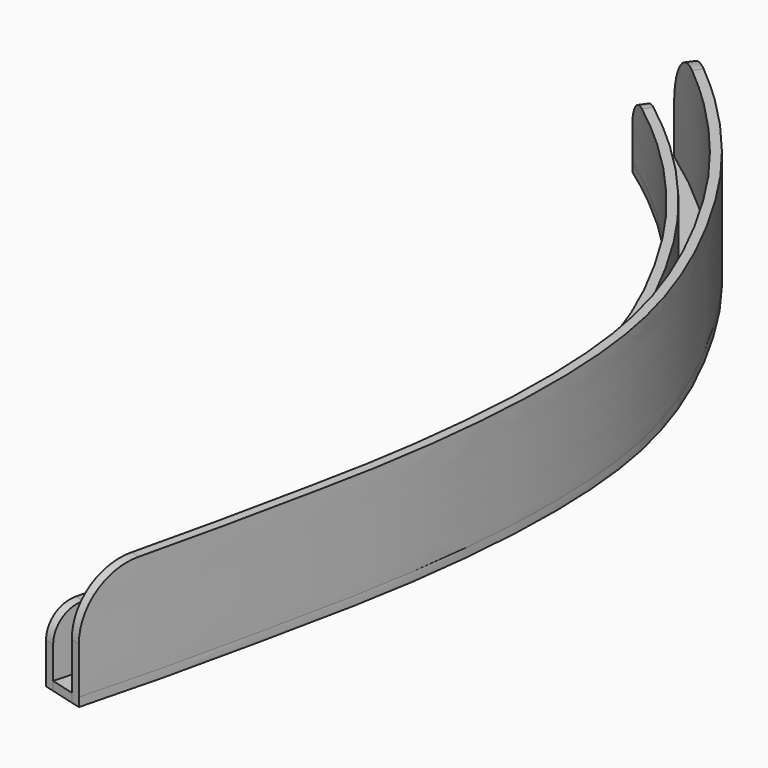
from build123d import *

# Parameters (mm, degrees)
F1_DEPTH = 1.5
F2_DEPTH = 12
F3_DEPTH = 19.5
F4_R     = 5
F5_R     = 10


# Not quite as in the source:
# - the dataset's text gives a spline's control points without its knots; the knots are read off the source's solid


with BuildPart() as f1:
    # F0 (on Top) → F1 (new body)
    with BuildSketch(Plane.XY):
        with BuildLine():
            Line((-5.5994206801, 1.5121137679), (-4.0547529063, 1.0949789353))
            add(Edge.make_bspline(
                [(-4.0547529063, 1.0949789353), (-2.7584482404, 5.8952494629), (-0.507776567, 14.8690865032), (1.6924327705, 24.7406730259), (3.2274659258, 31.9644086425), (4.3072829593, 37.0843203018), (5.3299777431, 41.9138704286), (6.2857824418, 46.6537900391), (7.0272963269, 50.6976340906), (7.5873908522, 54.0943139859), (7.9908458474, 56.7487025574), (8.3776794398, 59.5373035181), (8.7470381673, 62.4820190039), (9.0884901288, 65.5597847369), (9.4935897179, 69.8161894419), (9.8812175689, 75.3734994318), (10.0786737767, 82.263177237), (9.9568653112, 88.0547624157), (9.6514350357, 92.6366085021), (9.3098136977, 96.0260880656), (8.8477649235, 99.3496211049), (8.2569195036, 102.5793684142), (7.5320301271, 105.7399534193), (6.4089069299, 109.8549418842), (4.7452423063, 114.7999787819), (2.4491955615, 120.3732711408), (0.3841711701, 124.6808678941), (-1.2995078927, 127.9041144647), (-2.5628466606, 130.2043090367), (-3.8134120185, 132.3855904729), (-5.0303692601, 134.4303909952), (-6.225751369, 136.3562424102), (-7.8102832693, 138.7970536423), (-9.4097420041, 141.0929548178), (-11.0855205079, 143.3377393291), (-12.3960339805, 145.0187641433), (-13.7763443543, 146.7201318409), (-15.72650292, 149.0430807319), (-18.3677148559, 152.0208171993), (-21.9677844701, 155.7272991211), (-27.4687288943, 160.8505391151), (-32.5300323602, 164.9012591785), (-36.4483448757, 167.6911563366)],
                knots=[0, 0, 0, 0, 0.0625, 0.125, 0.15625, 0.1875, 0.21875, 0.25, 0.28125, 0.296875, 0.3125, 0.328125, 0.34375, 0.359375, 0.375, 0.40625, 0.4375, 0.46875, 0.484375, 0.5, 0.515625, 0.53125, 0.546875, 0.5625, 0.59375, 0.625, 0.65625, 0.671875, 0.6875, 0.703125, 0.71875, 0.734375, 0.75, 0.78125, 0.796875, 0.8125, 0.828125, 0.84375, 0.875, 0.90625, 0.9375, 1, 1, 1, 1], degree=3))
            Line((-36.4483448757, 167.6911563366), (-37.3763651787, 166.3877844337))
            add(Edge.make_bspline(
                [(-5.5994206801, 1.5121137679), (-4.3077783691, 6.2951193997), (-2.6258306552, 13.0012722172), (-0.7487467422, 21.1428564548), (0.5120539371, 26.8835227425), (1.6618421424, 32.2942963304), (2.7421119556, 37.4163284129), (3.763711516, 42.2407810647), (4.7148473297, 46.957842903), (5.4512317261, 50.973867239), (6.0070554882, 54.3446698739), (6.4074062474, 56.9786211877), (6.7913909073, 59.7466701592), (7.1580594369, 62.6699482968), (7.4968679186, 65.7239423227), (7.8986708212, 69.9457663896), (8.2827863792, 75.4536557983), (8.4780584917, 82.2716892525), (8.3575613015, 87.9906565389), (8.0566182326, 92.5041987263), (7.7206413282, 95.8370668347), (7.2673362217, 99.0969692413), (6.6893645236, 102.2561266917), (5.9799138442, 105.3495938294), (4.8790699069, 109.3831785269), (3.2460371404, 114.2377292155), (0.9873722214, 119.7207845936), (-1.0479591133, 123.9666951238), (-2.7098338186, 127.1482330689), (-3.9579699642, 129.4207865652), (-5.1952414945, 131.578886851), (-6.3982341438, 133.6001882211), (-7.5769680108, 135.4991721914), (-9.137149923, 137.90242787), (-10.7091151944, 140.1588272478), (-12.3574452199, 142.3668701842), (-13.6477758322, 144.0220399555), (-15.010114653, 145.7012846996), (-16.4552376121, 147.422652176), (-17.9785130359, 149.1706475813), (-20.1319914125, 151.5406139455), (-23.0870853339, 154.5830386116), (-28.5072460687, 159.6311117942), (-33.5019044586, 163.6291104104), (-37.3763651787, 166.3877844337)],
                knots=[0, 0, 0, 0, 0.0625, 0.09375, 0.125, 0.15625, 0.1875, 0.21875, 0.25, 0.28125, 0.296875, 0.3125, 0.328125, 0.34375, 0.359375, 0.375, 0.40625, 0.4375, 0.46875, 0.484375, 0.5, 0.515625, 0.53125, 0.546875, 0.5625, 0.59375, 0.625, 0.65625, 0.671875, 0.6875, 0.703125, 0.71875, 0.734375, 0.75, 0.78125, 0.796875, 0.8125, 0.828125, 0.84375, 0.859375, 0.875, 0.90625, 0.9375, 1, 1, 1, 1], degree=3))
        make_face()
        with BuildLine():
            Line((-4.0547529063, 1.0949789353), (0, 0))
            add(Edge.make_bspline(
                [(0, 0), (3.7575578317, 13.9143941924), (8.0227826013, 34.5697242327), (13.2830483989, 58.810255219), (16.3286613818, 102.3745951935), (0.7414565413, 134.1840402305), (-10.850321997, 150.6677651162), (-23.166189723, 163.3899207212), (-34.0122915804, 171.1125075817)],
                knots=[0, 0, 0, 0, 0.179472721, 0.3278596656, 0.5244539041, 0.7009046035, 0.8319408255, 1, 1, 1, 1], degree=3))
            Line((-34.0122915804, 171.1125075817), (-36.4483448757, 167.6911563366))
            add(Edge.make_bspline(
                [(-4.0547529063, 1.0949789353), (-2.7584482404, 5.8952494629), (-0.507776567, 14.8690865032), (1.6924327705, 24.7406730259), (3.2274659258, 31.9644086425), (4.3072829593, 37.0843203018), (5.3299777431, 41.9138704286), (6.2857824418, 46.6537900391), (7.0272963269, 50.6976340906), (7.5873908522, 54.0943139859), (7.9908458474, 56.7487025574), (8.3776794398, 59.5373035181), (8.7470381673, 62.4820190039), (9.0884901288, 65.5597847369), (9.4935897179, 69.8161894419), (9.8812175689, 75.3734994318), (10.0786737767, 82.263177237), (9.9568653112, 88.0547624157), (9.6514350357, 92.6366085021), (9.3098136977, 96.0260880656), (8.8477649235, 99.3496211049), (8.2569195036, 102.5793684142), (7.5320301271, 105.7399534193), (6.4089069299, 109.8549418842), (4.7452423063, 114.7999787819), (2.4491955615, 120.3732711408), (0.3841711701, 124.6808678941), (-1.2995078927, 127.9041144647), (-2.5628466606, 130.2043090367), (-3.8134120185, 132.3855904729), (-5.0303692601, 134.4303909952), (-6.225751369, 136.3562424102), (-7.8102832693, 138.7970536423), (-9.4097420041, 141.0929548178), (-11.0855205079, 143.3377393291), (-12.3960339805, 145.0187641433), (-13.7763443543, 146.7201318409), (-15.72650292, 149.0430807319), (-18.3677148559, 152.0208171993), (-21.9677844701, 155.7272991211), (-27.4687288943, 160.8505391151), (-32.5300323602, 164.9012591785), (-36.4483448757, 167.6911563366)],
                knots=[0, 0, 0, 0, 0.0625, 0.125, 0.15625, 0.1875, 0.21875, 0.25, 0.28125, 0.296875, 0.3125, 0.328125, 0.34375, 0.359375, 0.375, 0.40625, 0.4375, 0.46875, 0.484375, 0.5, 0.515625, 0.53125, 0.546875, 0.5625, 0.59375, 0.625, 0.65625, 0.671875, 0.6875, 0.703125, 0.71875, 0.734375, 0.75, 0.78125, 0.796875, 0.8125, 0.828125, 0.84375, 0.875, 0.90625, 0.9375, 1, 1, 1, 1], degree=3))
        make_face()
        with BuildLine():
            add(Edge.make_bspline(
                [(0, 0), (3.7575578317, 13.9143941924), (8.0227826013, 34.5697242327), (13.2830483989, 58.810255219), (16.3286613818, 102.3745951935), (0.7414565413, 134.1840402305), (-10.850321997, 150.6677651162), (-23.166189723, 163.3899207212), (-34.0122915804, 171.1125075817)],
                knots=[0, 0, 0, 0, 0.179472721, 0.3278596656, 0.5244539041, 0.7009046035, 0.8319408255, 1, 1, 1, 1], degree=3))
            Line((0, 0), (1.5446677738, -0.4171348325))
            add(Edge.make_bspline(
                [(1.5446677738, -0.4171348325), (2.8578698545, 4.4457075304), (4.5679258972, 11.2639826029), (6.471208409, 19.5204035077), (7.7459222074, 25.3246274254), (8.710660296, 29.861752913), (9.4415709252, 33.3270743816), (10.1516526278, 36.6841034318), (11.0080511968, 40.7313541909), (11.9802844095, 45.5506967156), (12.740553, 49.6964328886), (13.3161015114, 53.1867412996), (13.7308169961, 55.9152658826), (14.1279698827, 58.7783077194), (14.5070895277, 61.8008033997), (14.858119572, 64.964704693), (15.2751700405, 69.346464847), (15.675534421, 75.082961489), (15.880890085, 82.2322107178), (15.7290821349, 89.4984020152), (15.2348943815, 95.5282583731), (14.5771700718, 100.2636009959), (13.7259353942, 104.916437329), (12.3089473796, 110.5111606995), (10.1800206622, 116.8379202953), (7.7482745651, 122.7385719693), (5.5755901676, 127.2698429896), (3.813008393, 130.6440331992), (2.494237404, 133.0449928628), (1.1961735601, 135.3091193814), (-0.4949154505, 138.150738371), (-2.5759704926, 141.4308172445), (-5.1239386301, 145.0884119423), (-7.3757556815, 148.0369102178), (-9.3047861668, 150.4144945914), (-11.3377440532, 152.8360847708), (-14.1151484833, 155.9679162031), (-17.91014061, 159.8750407531), (-23.70432623, 165.271178621), (-29.0067696559, 169.5126373004), (-33.0842712775, 172.4158794846)],
                knots=[0, 0, 0, 0, 0.0625, 0.09375, 0.125, 0.15625, 0.171875, 0.1875, 0.21875, 0.25, 0.28125, 0.296875, 0.3125, 0.328125, 0.34375, 0.359375, 0.375, 0.40625, 0.4375, 0.46875, 0.5, 0.515625, 0.53125, 0.5625, 0.59375, 0.625, 0.65625, 0.671875, 0.6875, 0.703125, 0.71875, 0.75, 0.78125, 0.8125, 0.828125, 0.84375, 0.875, 0.90625, 0.9375, 1, 1, 1, 1], degree=3))
            Line((-33.0842712775, 172.4158794846), (-34.0122915804, 171.1125075817))
        make_face()
    extrude(amount=F1_DEPTH)

    # F0 (on Top) → F2 (join)
    with BuildSketch(Plane.XY):
        with BuildLine():
            Line((-5.5994206801, 1.5121137679), (-4.0547529063, 1.0949789353))
            add(Edge.make_bspline(
                [(-4.0547529063, 1.0949789353), (-2.7584482404, 5.8952494629), (-0.507776567, 14.8690865032), (1.6924327705, 24.7406730259), (3.2274659258, 31.9644086425), (4.3072829593, 37.0843203018), (5.3299777431, 41.9138704286), (6.2857824418, 46.6537900391), (7.0272963269, 50.6976340906), (7.5873908522, 54.0943139859), (7.9908458474, 56.7487025574), (8.3776794398, 59.5373035181), (8.7470381673, 62.4820190039), (9.0884901288, 65.5597847369), (9.4935897179, 69.8161894419), (9.8812175689, 75.3734994318), (10.0786737767, 82.263177237), (9.9568653112, 88.0547624157), (9.6514350357, 92.6366085021), (9.3098136977, 96.0260880656), (8.8477649235, 99.3496211049), (8.2569195036, 102.5793684142), (7.5320301271, 105.7399534193), (6.4089069299, 109.8549418842), (4.7452423063, 114.7999787819), (2.4491955615, 120.3732711408), (0.3841711701, 124.6808678941), (-1.2995078927, 127.9041144647), (-2.5628466606, 130.2043090367), (-3.8134120185, 132.3855904729), (-5.0303692601, 134.4303909952), (-6.225751369, 136.3562424102), (-7.8102832693, 138.7970536423), (-9.4097420041, 141.0929548178), (-11.0855205079, 143.3377393291), (-12.3960339805, 145.0187641433), (-13.7763443543, 146.7201318409), (-15.72650292, 149.0430807319), (-18.3677148559, 152.0208171993), (-21.9677844701, 155.7272991211), (-27.4687288943, 160.8505391151), (-32.5300323602, 164.9012591785), (-36.4483448757, 167.6911563366)],
                knots=[0, 0, 0, 0, 0.0625, 0.125, 0.15625, 0.1875, 0.21875, 0.25, 0.28125, 0.296875, 0.3125, 0.328125, 0.34375, 0.359375, 0.375, 0.40625, 0.4375, 0.46875, 0.484375, 0.5, 0.515625, 0.53125, 0.546875, 0.5625, 0.59375, 0.625, 0.65625, 0.671875, 0.6875, 0.703125, 0.71875, 0.734375, 0.75, 0.78125, 0.796875, 0.8125, 0.828125, 0.84375, 0.875, 0.90625, 0.9375, 1, 1, 1, 1], degree=3))
            Line((-36.4483448757, 167.6911563366), (-37.3763651787, 166.3877844337))
            add(Edge.make_bspline(
                [(-5.5994206801, 1.5121137679), (-4.3077783691, 6.2951193997), (-2.6258306552, 13.0012722172), (-0.7487467422, 21.1428564548), (0.5120539371, 26.8835227425), (1.6618421424, 32.2942963304), (2.7421119556, 37.4163284129), (3.763711516, 42.2407810647), (4.7148473297, 46.957842903), (5.4512317261, 50.973867239), (6.0070554882, 54.3446698739), (6.4074062474, 56.9786211877), (6.7913909073, 59.7466701592), (7.1580594369, 62.6699482968), (7.4968679186, 65.7239423227), (7.8986708212, 69.9457663896), (8.2827863792, 75.4536557983), (8.4780584917, 82.2716892525), (8.3575613015, 87.9906565389), (8.0566182326, 92.5041987263), (7.7206413282, 95.8370668347), (7.2673362217, 99.0969692413), (6.6893645236, 102.2561266917), (5.9799138442, 105.3495938294), (4.8790699069, 109.3831785269), (3.2460371404, 114.2377292155), (0.9873722214, 119.7207845936), (-1.0479591133, 123.9666951238), (-2.7098338186, 127.1482330689), (-3.9579699642, 129.4207865652), (-5.1952414945, 131.578886851), (-6.3982341438, 133.6001882211), (-7.5769680108, 135.4991721914), (-9.137149923, 137.90242787), (-10.7091151944, 140.1588272478), (-12.3574452199, 142.3668701842), (-13.6477758322, 144.0220399555), (-15.010114653, 145.7012846996), (-16.4552376121, 147.422652176), (-17.9785130359, 149.1706475813), (-20.1319914125, 151.5406139455), (-23.0870853339, 154.5830386116), (-28.5072460687, 159.6311117942), (-33.5019044586, 163.6291104104), (-37.3763651787, 166.3877844337)],
                knots=[0, 0, 0, 0, 0.0625, 0.09375, 0.125, 0.15625, 0.1875, 0.21875, 0.25, 0.28125, 0.296875, 0.3125, 0.328125, 0.34375, 0.359375, 0.375, 0.40625, 0.4375, 0.46875, 0.484375, 0.5, 0.515625, 0.53125, 0.546875, 0.5625, 0.59375, 0.625, 0.65625, 0.671875, 0.6875, 0.703125, 0.71875, 0.734375, 0.75, 0.78125, 0.796875, 0.8125, 0.828125, 0.84375, 0.859375, 0.875, 0.90625, 0.9375, 1, 1, 1, 1], degree=3))
        make_face()
    extrude(amount=F2_DEPTH)

    # F0 (on Top) → F3 (join)
    with BuildSketch(Plane.XY):
        with BuildLine():
            add(Edge.make_bspline(
                [(0, 0), (3.7575578317, 13.9143941924), (8.0227826013, 34.5697242327), (13.2830483989, 58.810255219), (16.3286613818, 102.3745951935), (0.7414565413, 134.1840402305), (-10.850321997, 150.6677651162), (-23.166189723, 163.3899207212), (-34.0122915804, 171.1125075817)],
                knots=[0, 0, 0, 0, 0.179472721, 0.3278596656, 0.5244539041, 0.7009046035, 0.8319408255, 1, 1, 1, 1], degree=3))
            Line((0, 0), (1.5446677738, -0.4171348325))
            add(Edge.make_bspline(
                [(1.5446677738, -0.4171348325), (2.8578698545, 4.4457075304), (4.5679258972, 11.2639826029), (6.471208409, 19.5204035077), (7.7459222074, 25.3246274254), (8.710660296, 29.861752913), (9.4415709252, 33.3270743816), (10.1516526278, 36.6841034318), (11.0080511968, 40.7313541909), (11.9802844095, 45.5506967156), (12.740553, 49.6964328886), (13.3161015114, 53.1867412996), (13.7308169961, 55.9152658826), (14.1279698827, 58.7783077194), (14.5070895277, 61.8008033997), (14.858119572, 64.964704693), (15.2751700405, 69.346464847), (15.675534421, 75.082961489), (15.880890085, 82.2322107178), (15.7290821349, 89.4984020152), (15.2348943815, 95.5282583731), (14.5771700718, 100.2636009959), (13.7259353942, 104.916437329), (12.3089473796, 110.5111606995), (10.1800206622, 116.8379202953), (7.7482745651, 122.7385719693), (5.5755901676, 127.2698429896), (3.813008393, 130.6440331992), (2.494237404, 133.0449928628), (1.1961735601, 135.3091193814), (-0.4949154505, 138.150738371), (-2.5759704926, 141.4308172445), (-5.1239386301, 145.0884119423), (-7.3757556815, 148.0369102178), (-9.3047861668, 150.4144945914), (-11.3377440532, 152.8360847708), (-14.1151484833, 155.9679162031), (-17.91014061, 159.8750407531), (-23.70432623, 165.271178621), (-29.0067696559, 169.5126373004), (-33.0842712775, 172.4158794846)],
                knots=[0, 0, 0, 0, 0.0625, 0.09375, 0.125, 0.15625, 0.171875, 0.1875, 0.21875, 0.25, 0.28125, 0.296875, 0.3125, 0.328125, 0.34375, 0.359375, 0.375, 0.40625, 0.4375, 0.46875, 0.5, 0.515625, 0.53125, 0.5625, 0.59375, 0.625, 0.65625, 0.671875, 0.6875, 0.703125, 0.71875, 0.75, 0.78125, 0.8125, 0.828125, 0.84375, 0.875, 0.90625, 0.9375, 1, 1, 1, 1], degree=3))
            Line((-33.0842712775, 172.4158794846), (-34.0122915804, 171.1125075817))
        make_face()
    extrude(amount=F3_DEPTH)

    # F4
    f4_edges = [f1.edges().sort_by_distance(p)[0] for p in [
        (-36.912355, 167.03947, 12),
        (-4.827087, 1.303546, 12),
    ]]
    fillet(f4_edges, radius=F4_R)

    # F5
    f5_edges = [f1.edges().sort_by_distance(p)[0] for p in [
        (-33.548281, 171.764194, 19.5),
        (0.772334, -0.208567, 19.5),
    ]]
    fillet(f5_edges, radius=F5_R)


solid = f1.part
